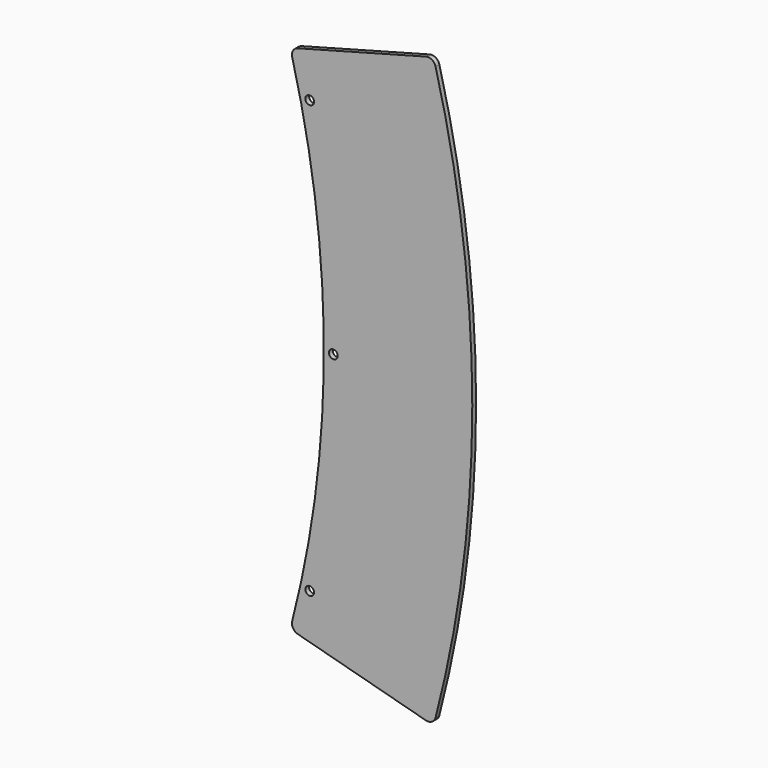
from build123d import *

# Parameters (mm, degrees)
F2_DEPTH        = 3
F4_D            = 5.5
F4_COPIES_COUNT = 3
F4_COPIES_ANGLE = 25
F5_R            = 5


# Not quite as in the source:
# - a pattern or mirror of a feature is missing from the dataset's text; its kind, count and spacing are read off the source's solid


with BuildPart() as f2:
    # F1 (on Front) → F2 (new body)
    with BuildSketch(Plane.XZ):
        with BuildLine():
            Line((604.669567257, -162.0207222342), (695.4665949281, -186.3497124738))
            ThreePointArc((695.4665949281, -186.3497124738), (720, 0), (695.4665949281, 186.3497124738))
            Line((695.4665949281, 186.3497124738), (604.669567257, 162.0207222342))
            ThreePointArc((604.669567257, 162.0207222342), (626, 0), (604.669567257, -162.0207222342))
        make_face()
    extrude(amount=-F2_DEPTH)

    # F4 (through all)
    with Locations(Plane.XZ):
        with Locations((617.0190764998, -136.7898360089)):
            f4 = Hole(F4_D / 2)

    # F4_copies: F4 ×3 about axis
    f4_copies_axis = Axis((0, 0, 0), (0, -1, 0))
    for i in range(1, F4_COPIES_COUNT):
        add(f4.rotate(f4_copies_axis, i * F4_COPIES_ANGLE / (F4_COPIES_COUNT - 1)), mode=Mode.SUBTRACT)

    # F5
    f5_edges = [f2.edges().sort_by_distance(p)[0] for p in [
        (695.466595, 1.5, 186.349712),
        (604.669567, 1.5, 162.020722),
        (695.466595, 1.5, -186.349712),
        (604.669567, 1.5, -162.020722),
    ]]
    fillet(f5_edges, radius=F5_R)


solid = f2.part
